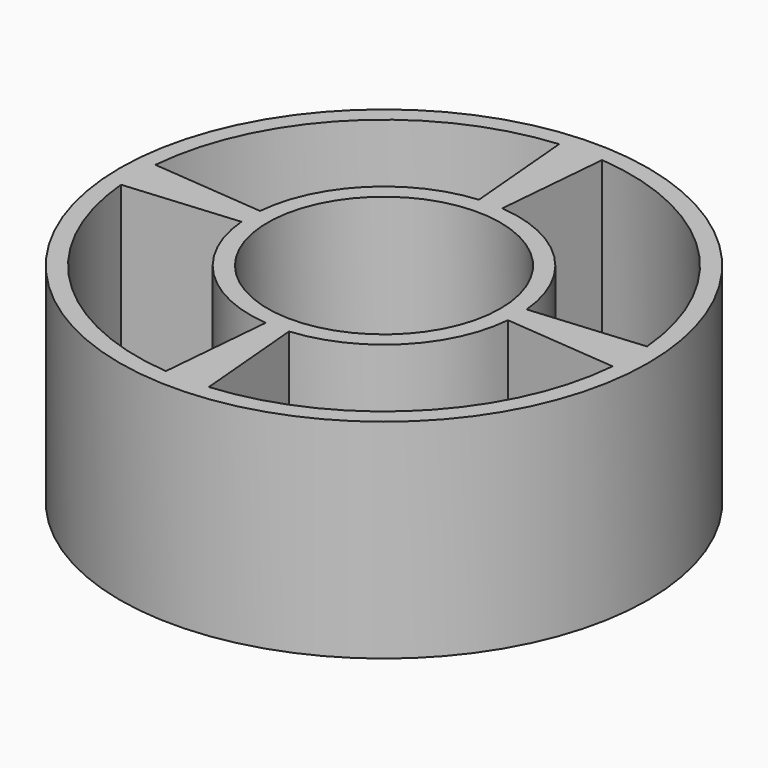
from build123d import *

# Parameters (mm, degrees)
F0_R         = 38
F1_DEPTH     = 30
F2_R         = 16.75
F3_DEPTH     = 22
F4_TEXT_SIZE = 15.0948482092
F5_DEPTH     = 2


# Not quite as in the source:
# - Text() gives the source's letters only with a copy of the font that has no kerning and outlines rounded to 1/6400 em; it was checked with that copy


with BuildPart() as f1:
    # F0 (on Top) → F1 (new body)
    with BuildSketch(Plane.XY):
        Circle(F0_R)
    extrude(amount=F1_DEPTH)

    # F2 (on face) → F3 (cut)
    with BuildSketch(Plane.XY.offset(30)):
        with BuildLine():
            Line((-1.6777480479, 19.1767479383), (-3.0940288675, 35.3649117823))
            ThreePointArc((-3.0940288675, 35.3649117823), (-25.1022907321, 25.1022907321), (-35.3649117823, 3.0940288675))
            Line((-35.3649117823, 3.0940288675), (-19.1767479383, 1.6777480479))
            ThreePointArc((-19.1767479383, 1.6777480479), (-13.6118055378, 13.6118055378), (-1.6777480479, 19.1767479383))
        make_face()
        with BuildLine():
            Line((3.0940288675, 35.3649117823), (1.6777480479, 19.1767479383))
            ThreePointArc((1.6777480479, 19.1767479383), (13.6118055378, 13.6118055378), (19.1767479383, 1.6777480479))
            Line((19.1767479383, 1.6777480479), (35.3649117823, 3.0940288675))
            ThreePointArc((35.3649117823, 3.0940288675), (25.1022907321, 25.1022907321), (3.0940288675, 35.3649117823))
        make_face()
        with BuildLine():
            ThreePointArc((-1.6777480479, -19.1767479383), (-13.6118055378, -13.6118055378), (-19.1767479383, -1.6777480479))
            Line((-19.1767479383, -1.6777480479), (-35.3649117823, -3.0940288675))
            ThreePointArc((-35.3649117823, -3.0940288675), (-25.1022907321, -25.1022907321), (-3.0940288675, -35.3649117823))
            Line((-3.0940288675, -35.3649117823), (-1.6777480479, -19.1767479383))
        make_face()
        with BuildLine():
            Line((1.6777480479, -19.1767479383), (3.0940288675, -35.3649117823))
            ThreePointArc((3.0940288675, -35.3649117823), (25.1022907321, -25.1022907321), (35.3649117823, -3.0940288675))
            Line((35.3649117823, -3.0940288675), (19.1767479383, -1.6777480479))
            ThreePointArc((19.1767479383, -1.6777480479), (13.6118055378, -13.6118055378), (1.6777480479, -19.1767479383))
        make_face()
        Circle(F2_R)
    extrude(amount=-F3_DEPTH, mode=Mode.SUBTRACT)

    # F4 (on face) → F5 (cut)
    with BuildSketch(Plane(origin=(0, 0, 0), x_dir=(1, 0, 0), z_dir=(0, 0, -1))):
        with Locations((-34.8796120487, -5.2811949803)):
            Text('Footbutts', F4_TEXT_SIZE, font='Arimo', font_style=FontStyle.BOLD, text_align=(TextAlign.LEFT, TextAlign.BOTTOM))
    extrude(amount=-F5_DEPTH, mode=Mode.SUBTRACT)


solid = f1.part
